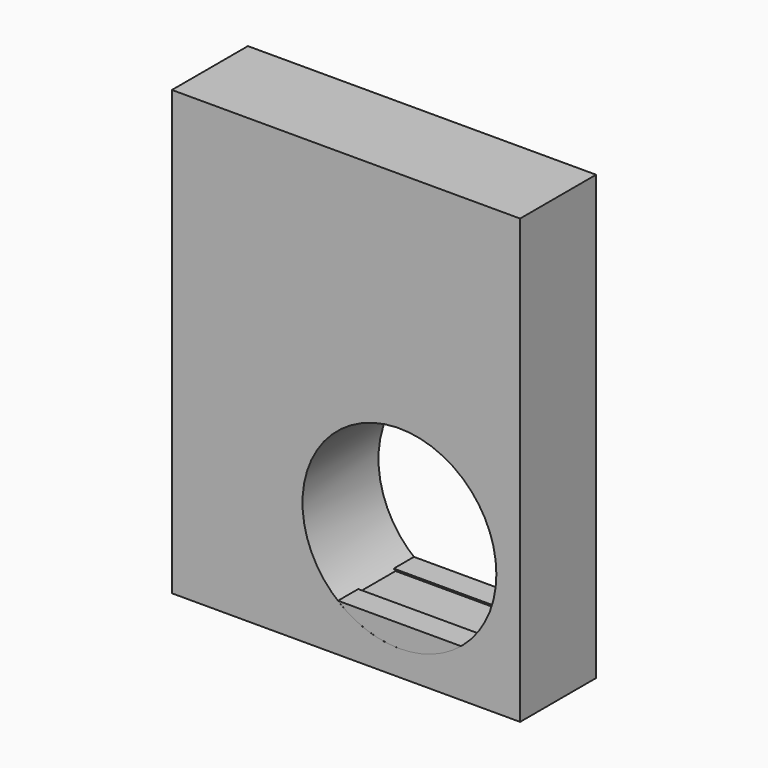
from build123d import *

# Parameters (mm, degrees)
F0_W     = 279.4
F0_H     = 355.6
F1_DEPTH = 38.1
F2_R     = 77.7875
F3_DEPTH = 76.201
F5_DEPTH = 76.2
F6_W     = 98.9948503711
F6_H     = 35.56
F7_DEPTH = 1.27


with BuildPart() as f1:
    # F0 (on Front) → F1 (new body, symmetric)
    with BuildSketch(Plane.XZ):
        with Locations((139.7, 177.8)):
            Rectangle(F0_W, F0_H)
    extrude(amount=F1_DEPTH, both=True)

    # F2 (on face) → F3 (cut, through all)
    with BuildSketch(Plane.XZ.offset(38.1)):
        with Locations((182.5625, 98.1075)):
            Circle(F2_R)
    extrude(amount=-F3_DEPTH, mode=Mode.SUBTRACT)


with BuildPart() as f5:
    # F4 (on face) → F5 (new body, through all)
    with BuildSketch(Plane.XZ.offset(38.1)):
        with BuildLine():
            Line((182.5625, 38.1), (133.0650748144, 38.1))
            ThreePointArc((133.0650748144, 38.1), (182.5625, 20.32), (232.0599251856, 38.1))
            Line((232.0599251856, 38.1), (182.5625, 38.1))
        make_face()
    extrude(amount=-F5_DEPTH)

    # F6 (on face) → F7 (cut)
    with BuildSketch(Plane.XY.offset(38.1)):
        with Locations((182.5625, 0)):
            Rectangle(F6_W, F6_H)
    extrude(amount=-F7_DEPTH, mode=Mode.SUBTRACT)


solid = Compound([f1.part, f5.part])
